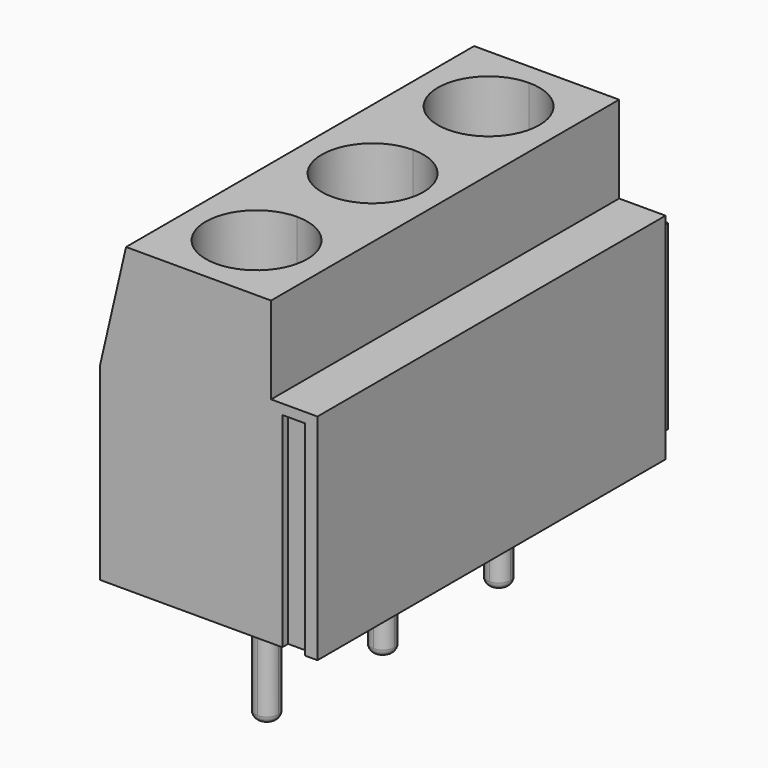
from build123d import *

# Parameters (mm, degrees)
F1_DEPTH  = 15
F3_DEPTH  = 3
F4_W      = 0.5
F4_H      = 0.5
F5_DEPTH  = 0.5
F6_DEPTH  = 1.3
F7_DEPTH  = 3.3
F8_SIZE   = 1
F9_W      = 0.7894294686
F9_H      = 7.0516658016
F10_DEPTH = 0.25
F11_W     = 0.5
F11_H     = 6.2580032973
F12_DEPTH = 0.5
F14_DEPTH = 4
F6_FACE_W = 1
F6_FACE_H = 0.5
F16_DEPTH = 2.6


# Not quite as in the source:
# - a fillet or chamfer that OpenCascade refuses, or shapes differently, is made with other operations: its cross-section is extruded or revolved along the edge and cut away or added


with BuildPart() as f1:
    # F0 (on Front) → F1 (new body)
    with BuildSketch(Plane.XZ):
        Polygon((-7.5, 0), (0, 0), (0, 7.397435054), (-1.6, 7.397435054), (-1.6, 10.397435054), (-6.6, 10.397435054), (-7.5, 6.5), align=None)
    extrude(amount=F1_DEPTH)

    # F2 (on face) → F3 (cut)
    with BuildSketch(Plane.XY.offset(10.397435054)):
        with BuildLine():
            ThreePointArc((-2.35, -2.5), (-2.8625631329, -1.2625631329), (-4.1, -0.75))
            Line((-4.1, -0.75), (-4.1, -2.5))
            Line((-4.1, -2.5), (-4.1, -4.25))
            ThreePointArc((-4.1, -4.25), (-2.8625631329, -3.7374368671), (-2.35, -2.5))
        make_face()
        with BuildLine():
            ThreePointArc((-2.35, -12.5), (-2.8625631329, -11.2625631329), (-4.1, -10.75))
            Line((-4.1, -10.75), (-4.1, -14.25))
            ThreePointArc((-4.1, -14.25), (-2.8625631329, -13.7374368671), (-2.35, -12.5))
        make_face()
        with BuildLine():
            Line((-4.1, -14.25), (-4.1, -10.75))
            ThreePointArc((-4.1, -10.75), (-5.85, -12.5), (-4.1, -14.25))
        make_face()
        with BuildLine():
            ThreePointArc((-2.35, -7.5), (-2.8625631329, -6.2625631329), (-4.1, -5.75))
            Line((-4.1, -5.75), (-4.1, -7.5))
            Line((-4.1, -7.5), (-2.35, -7.5))
        make_face()
        with BuildLine():
            Line((-4.1, -7.5), (-4.1, -5.75))
            ThreePointArc((-4.1, -5.75), (-5.85, -7.5), (-4.1, -9.25))
            Line((-4.1, -9.25), (-4.1, -7.5))
        make_face()
        with BuildLine():
            Line((-4.1, -2.5), (-4.1, -0.75))
            ThreePointArc((-4.1, -0.75), (-5.85, -2.5), (-4.1, -4.25))
            Line((-4.1, -4.25), (-4.1, -2.5))
        make_face()
        with BuildLine():
            Line((-2.35, -7.5), (-4.1, -7.5))
            Line((-4.1, -7.5), (-4.1, -9.25))
            ThreePointArc((-4.1, -9.25), (-2.8625631329, -8.7374368671), (-2.35, -7.5))
        make_face()
    extrude(amount=-F3_DEPTH, mode=Mode.SUBTRACT)

    # F4 (on face) → F5 (cut)
    with BuildSketch(Plane(origin=(-7.5, 0, 0), x_dir=(0, -1, 0), z_dir=(-1, 0, 0))):
        with Locations((2.510879118, 0.25)):
            Rectangle(F4_W, F4_H)
        with Locations((12.510879118, 0.25)):
            Rectangle(F4_W, F4_H)
        with Locations((7.510879118, 0.25)):
            Rectangle(F4_W, F4_H)
        with Locations((3.010879118, 0.25)):
            Rectangle(F4_W, F4_H)
        Polygon((0.760879118, 0.5), (2.260879118, 0.5), (2.760879118, 0.5), (2.760879118, 1), (1.260879118, 1), (1.260879118, 4.5), (0.760879118, 5.5), align=None)
        Polygon((2.760879118, 1), (2.760879118, 0.5), (3.260879118, 0.5), (4.760879118, 0.5), (4.760879118, 5.5), (4.260879118, 4.5), (4.260879118, 1), align=None)
        Polygon((0.760879118, 6), (0.760879118, 5.5), (1.260879118, 4.5), (1.760879118, 3.5), (2.760879118, 3.5), (2.760879118, 5.5), (2.760879118, 6), align=None)
        with Locations((8.010879118, 0.25)):
            Rectangle(F4_W, F4_H)
        Polygon((5.760879118, 0.5), (7.260879118, 0.5), (7.760879118, 0.5), (7.760879118, 1), (6.260879118, 1), (6.260879118, 4.5), (5.760879118, 5.5), align=None)
        Polygon((2.760879118, 5.5), (2.760879118, 3.5), (3.760879118, 3.5), (4.260879118, 4.5), (4.760879118, 5.5), (4.760879118, 6), (2.760879118, 6), align=None)
        Polygon((7.760879118, 1), (7.760879118, 0.5), (8.260879118, 0.5), (9.760879118, 0.5), (9.760879118, 5.5), (9.260879118, 4.5), (9.260879118, 1), align=None)
        Polygon((5.760879118, 6), (5.760879118, 5.5), (6.260879118, 4.5), (6.760879118, 3.5), (7.760879118, 3.5), (7.760879118, 5.5), (7.760879118, 6), align=None)
        with Locations((13.010879118, 0.25)):
            Rectangle(F4_W, F4_H)
        Polygon((10.760879118, 0.5), (12.260879118, 0.5), (12.760879118, 0.5), (12.760879118, 1), (11.260879118, 1), (11.260879118, 4.5), (10.760879118, 5.5), align=None)
        Polygon((7.760879118, 5.5), (7.760879118, 3.5), (8.760879118, 3.5), (9.260879118, 4.5), (9.760879118, 5.5), (9.760879118, 6), (7.760879118, 6), align=None)
        Polygon((12.760879118, 1), (12.760879118, 0.5), (13.260879118, 0.5), (14.760879118, 0.5), (14.760879118, 5.5), (14.260879118, 4.5), (14.260879118, 1), align=None)
        Polygon((10.760879118, 6), (10.760879118, 5.5), (11.260879118, 4.5), (11.760879118, 3.5), (12.760879118, 3.5), (12.760879118, 5.5), (12.760879118, 6), align=None)
        Polygon((12.760879118, 5.5), (12.760879118, 3.5), (13.760879118, 3.5), (14.260879118, 4.5), (14.760879118, 5.5), (14.760879118, 6), (12.760879118, 6), align=None)
        Polygon((1.260879118, 1), (2.760879118, 1), (2.760879118, 3.5), (1.760879118, 3.5), (1.260879118, 4.5), align=None)
        Polygon((2.760879118, 3.5), (2.760879118, 1), (4.260879118, 1), (4.260879118, 4.5), (3.760879118, 3.5), align=None)
        Polygon((6.260879118, 1), (7.760879118, 1), (7.760879118, 3.5), (6.760879118, 3.5), (6.260879118, 4.5), align=None)
        Polygon((7.760879118, 3.5), (7.760879118, 1), (9.260879118, 1), (9.260879118, 4.5), (8.760879118, 3.5), align=None)
        Polygon((11.260879118, 1), (12.760879118, 1), (12.760879118, 3.5), (11.760879118, 3.5), (11.260879118, 4.5), align=None)
        Polygon((12.760879118, 3.5), (12.760879118, 1), (14.260879118, 1), (14.260879118, 4.5), (13.760879118, 3.5), align=None)
    extrude(amount=-F5_DEPTH, mode=Mode.SUBTRACT)

    # F4 (on face) → F6 (cut)
    with BuildSketch(Plane(origin=(-7.5, 0, 0), x_dir=(0, -1, 0), z_dir=(-1, 0, 0))):
        Polygon((0.760879118, 0.5), (2.260879118, 0.5), (2.760879118, 0.5), (2.760879118, 1), (1.260879118, 1), (1.260879118, 4.5), (0.760879118, 5.5), align=None)
        Polygon((1.260879118, 1), (2.760879118, 1), (2.760879118, 3.5), (1.760879118, 3.5), (1.260879118, 4.5), align=None)
        Polygon((2.760879118, 3.5), (2.760879118, 1), (4.260879118, 1), (4.260879118, 4.5), (3.760879118, 3.5), align=None)
        Polygon((2.760879118, 1), (2.760879118, 0.5), (3.260879118, 0.5), (4.760879118, 0.5), (4.760879118, 5.5), (4.260879118, 4.5), (4.260879118, 1), align=None)
        Polygon((5.760879118, 0.5), (7.260879118, 0.5), (7.760879118, 0.5), (7.760879118, 1), (6.260879118, 1), (6.260879118, 4.5), (5.760879118, 5.5), align=None)
        Polygon((6.260879118, 1), (7.760879118, 1), (7.760879118, 3.5), (6.760879118, 3.5), (6.260879118, 4.5), align=None)
        Polygon((7.760879118, 3.5), (7.760879118, 1), (9.260879118, 1), (9.260879118, 4.5), (8.760879118, 3.5), align=None)
        Polygon((7.760879118, 1), (7.760879118, 0.5), (8.260879118, 0.5), (9.760879118, 0.5), (9.760879118, 5.5), (9.260879118, 4.5), (9.260879118, 1), align=None)
        Polygon((12.260879118, 0.5), (12.760879118, 0.5), (12.760879118, 1), (11.260879118, 1), (11.260879118, 4.5), (10.760879118, 5.5), (10.760879118, 0.5), align=None)
        Polygon((11.260879118, 1), (12.760879118, 1), (12.760879118, 3.5), (11.760879118, 3.5), (11.260879118, 4.5), align=None)
        Polygon((12.760879118, 3.5), (12.760879118, 1), (14.260879118, 1), (14.260879118, 4.5), (13.760879118, 3.5), align=None)
        Polygon((12.760879118, 0.5), (13.260879118, 0.5), (14.760879118, 0.5), (14.760879118, 5.5), (14.260879118, 4.5), (14.260879118, 1), (12.760879118, 1), align=None)
    extrude(amount=-F6_DEPTH, mode=Mode.SUBTRACT)

    # F4 (on face) → F7 (cut)
    with BuildSketch(Plane(origin=(-7.5, 0, 0), x_dir=(0, -1, 0), z_dir=(-1, 0, 0))):
        Polygon((1.260879118, 1), (2.760879118, 1), (2.760879118, 3.5), (1.760879118, 3.5), (1.260879118, 4.5), align=None)
        Polygon((2.760879118, 3.5), (2.760879118, 1), (4.260879118, 1), (4.260879118, 4.5), (3.760879118, 3.5), align=None)
        Polygon((6.260879118, 1), (7.760879118, 1), (7.760879118, 3.5), (6.760879118, 3.5), (6.260879118, 4.5), align=None)
        Polygon((7.760879118, 3.5), (7.760879118, 1), (9.260879118, 1), (9.260879118, 4.5), (8.760879118, 3.5), align=None)
        Polygon((11.260879118, 1), (12.760879118, 1), (12.760879118, 3.5), (11.760879118, 3.5), (11.260879118, 4.5), align=None)
        Polygon((12.760879118, 3.5), (12.760879118, 1), (14.260879118, 1), (14.260879118, 4.5), (13.760879118, 3.5), align=None)
    extrude(amount=-F7_DEPTH, mode=Mode.SUBTRACT)

    # F8
    f8_edges = [f1.edges().sort_by_distance(p)[0] for p in [
        (-7, -2.760879, 3.5),
        (-7, -7.760879, 3.5),
        (-7, -12.760879, 3.5),
    ]]
    chamfer(f8_edges, length=F8_SIZE)

    # F9 (on face) → F10 (cut)
    with BuildSketch(Plane.XZ.offset(15)):
        with Locations((-0.816616026, 3.5258329008)):
            Rectangle(F9_W, F9_H)
    extrude(amount=-F10_DEPTH, mode=Mode.SUBTRACT)

    # F11 (on face) → F12 (join)
    with BuildSketch(Plane(origin=(0, 0, 0), x_dir=(-1, 0, 0), z_dir=(0, 1, 0))):
        with Locations((0.5626286319, 3.7392643862)):
            Rectangle(F11_W, F11_H)
    extrude(amount=F12_DEPTH)

    # F13 (on face) → F14 (join)
    with BuildSketch(Plane(origin=(0, 0, 0), x_dir=(1, 0, 0), z_dir=(0, 0, -1))):
        with BuildLine():
            ThreePointArc((-3.35, 12.5), (-3.4671572875, 12.7828427125), (-3.75, 12.9))
            Line((-3.75, 12.9), (-3.75, 12.5))
            Line((-3.75, 12.5), (-3.75, 12.1))
            ThreePointArc((-3.75, 12.1), (-3.4671572875, 12.2171572875), (-3.35, 12.5))
        make_face()
        with BuildLine():
            ThreePointArc((-3.35, 2.5), (-3.4671572875, 2.7828427125), (-3.75, 2.9))
            Line((-3.75, 2.9), (-3.75, 2.1))
            ThreePointArc((-3.75, 2.1), (-3.4671572875, 2.2171572875), (-3.35, 2.5))
        make_face()
        with BuildLine():
            Line((-3.75, 2.1), (-3.75, 2.9))
            ThreePointArc((-3.75, 2.9), (-4.15, 2.5), (-3.75, 2.1))
        make_face()
        with BuildLine():
            ThreePointArc((-3.35, 7.5), (-3.4671572875, 7.7828427125), (-3.75, 7.9))
            Line((-3.75, 7.9), (-3.75, 7.5))
            Line((-3.75, 7.5), (-3.35, 7.5))
        make_face()
        with BuildLine():
            Line((-3.75, 7.5), (-3.75, 7.9))
            ThreePointArc((-3.75, 7.9), (-4.15, 7.5), (-3.75, 7.1))
            Line((-3.75, 7.1), (-3.75, 7.5))
        make_face()
        with BuildLine():
            Line((-3.75, 12.5), (-3.75, 12.9))
            ThreePointArc((-3.75, 12.9), (-4.15, 12.5), (-3.75, 12.1))
            Line((-3.75, 12.1), (-3.75, 12.5))
        make_face()
        with BuildLine():
            Line((-3.35, 7.5), (-3.75, 7.5))
            Line((-3.75, 7.5), (-3.75, 7.1))
            ThreePointArc((-3.75, 7.1), (-3.4671572875, 7.2171572875), (-3.35, 7.5))
        make_face()
    extrude(amount=F14_DEPTH)

    # F15: fillet of radius 0.25 on 3 edges, made by hand

    # F15_s1 → F15_t2 (revolve, cut)
    with BuildSketch(Plane.YZ.offset(-3.75)):
        with BuildLine():
            ThreePointArc((-12.9, -3.75), (-12.8267766953, -3.9267766953), (-12.65, -4))
            Line((-12.65, -4), (-12.9, -4))
            Line((-12.9, -4), (-12.9, -3.75))
        make_face()
    revolve(axis=Axis((-3.75, -12.5, -4), (0, 0, -1)), mode=Mode.SUBTRACT)

    # F15_s3 → F15_t4 (revolve, cut)
    with BuildSketch(Plane.YZ.offset(-3.75)):
        with BuildLine():
            ThreePointArc((-7.1, -3.75), (-7.1732233047, -3.9267766953), (-7.35, -4))
            Line((-7.35, -4), (-7.1, -4))
            Line((-7.1, -4), (-7.1, -3.75))
        make_face()
    revolve(axis=Axis((-3.75, -7.5, -4), (0, 0, -1)), mode=Mode.SUBTRACT)

    # F15_s5 → F15_t6 (revolve, cut)
    with BuildSketch(Plane.YZ.offset(-3.75)):
        with BuildLine():
            ThreePointArc((-2.9, -3.75), (-2.8267766953, -3.9267766953), (-2.65, -4))
            Line((-2.65, -4), (-2.9, -4))
            Line((-2.9, -4), (-2.9, -3.75))
        make_face()
    revolve(axis=Axis((-3.75, -2.5, -4), (0, 0, -1)), mode=Mode.SUBTRACT)

    # F6_face (on face) + F4 (on face) → F16 (cut)
    with BuildSketch(Plane(origin=(-7, -12.760879118, 0.25), x_dir=(0, -1, 0), z_dir=(-1, 0, 0))):
        Rectangle(F6_FACE_W, F6_FACE_H)
        with Locations((-5, 0)):
            Rectangle(F6_FACE_W, F6_FACE_H)
    with BuildSketch(Plane(origin=(-7.5, 0, 0), x_dir=(0, -1, 0), z_dir=(-1, 0, 0))):
        with Locations((3.010879118, 0.25)):
            Rectangle(F4_W, F4_H)
        with Locations((2.510879118, 0.25)):
            Rectangle(F4_W, F4_H)
    extrude(amount=-F16_DEPTH, mode=Mode.SUBTRACT)


solid = f1.part
